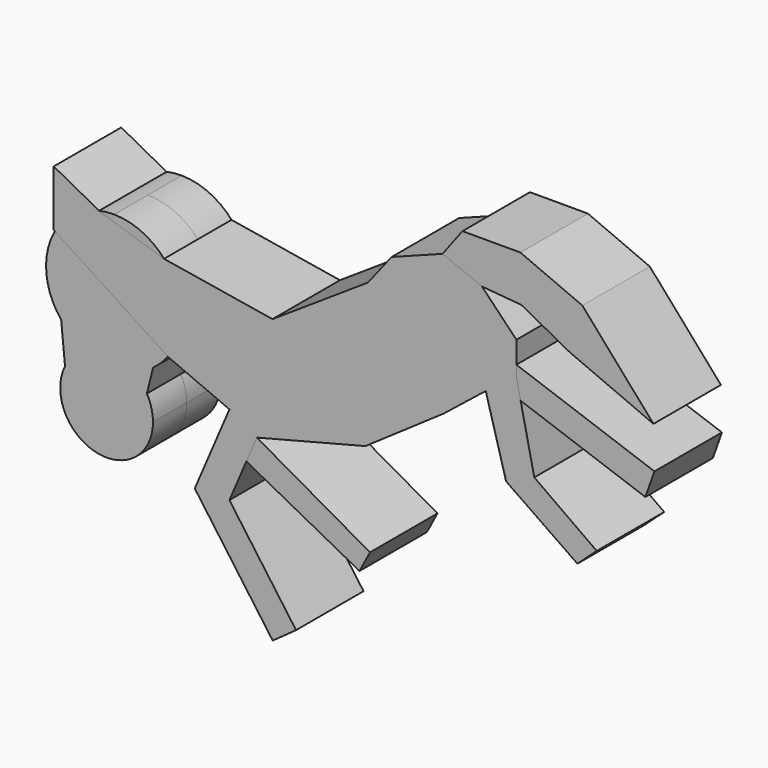
from build123d import *

# Parameters (mm, degrees)
F0_W        = 150.6141573191
F0_H        = 79.405464232
F1_DEPTH    = 63.5
F2_T1_DEPTH = 658.6141573191
F3_T1_DEPTH = 718.5752538832
F7_DEPTH    = 12.7
F9_DEPTH    = 12.7
F10_DEPTH   = 12.7


# Not quite as in the source:
# - a fillet or chamfer that OpenCascade refuses, or shapes differently, is made with other operations: its cross-section is extruded or revolved along the edge and cut away or added


with BuildPart() as f1:
    # F0 (on Front) → F1 (new body, symmetric)
    with BuildSketch(Plane.XZ):
        with Locations((-10.1514682174, 0)):
            Rectangle(F0_W, F0_H)
    extrude(amount=F1_DEPTH, both=True)

    # F2: fillet of radius 101.6 on 2 edges, made by hand

    # F2_s2 → F2_t1 (cut)
    with BuildSketch(Plane.YZ.offset(-339.4585468769)):
        with BuildLine():
            ThreePointArc((-38.1, -39.702732116), (33.7420489686, -9.9447810845), (63.5, 61.897267884))
            Line((63.5, 61.897267884), (63.5, -39.702732116))
            Line((63.5, -39.702732116), (-38.1, -39.702732116))
        make_face()
        with BuildLine():
            ThreePointArc((38.1, -39.702732116), (-33.7420489686, -9.9447810845), (-63.5, 61.897267884))
            Line((-63.5, 61.897267884), (-63.5, -39.702732116))
            Line((-63.5, -39.702732116), (38.1, -39.702732116))
        make_face()
    extrude(amount=F2_T1_DEPTH, mode=Mode.SUBTRACT)

    # F3: fillet of radius 63.5 on 1 edges, made by hand

    # F3_s2 → F3_t1 (cut)
    with BuildSketch(Plane.YZ.offset(-369.439095159)):
        with BuildLine():
            ThreePointArc((-63.5, 61.8972269458), (0, -1.6027474678), (63.5, 61.8972269458))
            ThreePointArc((63.5, 61.8972269458), (46.1422582324, 5.1011242834), (0, -32.2884529021))
            ThreePointArc((0, -32.2884529021), (-46.1422582324, 5.1011242834), (-63.5, 61.8972269458))
        make_face()
    extrude(amount=F3_T1_DEPTH, mode=Mode.SUBTRACT)


with BuildPart() as f1b:
    # F0 (on Front) → F1, piece 2 (new body, symmetric)
    with BuildSketch(Plane.XZ):
        Polygon((31.3350483775, 122.2248598933), (31.3350483775, 93.6296462137), (77.3309990764, 97.4231287837), (73.4557332426, 72.6213976741), (123.3269497752, 72.6213976741), (123.3269497752, 122.2248598933), align=None)
        Polygon((77.3309990764, 97.4231287837), (31.3350483775, 93.6296462137), (31.3350483775, 72.6213976741), (73.4557332426, 72.6213976741), align=None)
    extrude(amount=F1_DEPTH, both=True)


with BuildPart() as f7:
    # F6 (on Front) → F7 (new body, symmetric)
    with BuildSketch(Plane.XZ):
        with BuildLine():
            ThreePointArc((-36.6087691493, 35.5593333212), (-32.619344121, 34.8654693263), (-28.9966608866, 33.0562912025))
            ThreePointArc((-28.9966608866, 33.0562912025), (-25.8689313613, 34.2954979773), (-22.9885519546, 36.0338132212))
            Line((-22.9885519546, 36.0338132212), (-16.6514110853, 61.4541698217))
            ThreePointArc((-16.6514110853, 61.4541698217), (-24.0542736375, 69.6886763572), (-34.6755571583, 72.818821437))
            Line((-34.6755571583, 72.818821437), (-36.6087691493, 35.5593333212))
        make_face()
        with BuildLine():
            ThreePointArc((-43.3512285275, 34.0273458631), (-40.0763049725, 35.2171943654), (-36.6087691493, 35.5593333212))
            Line((-36.6087691493, 35.5593333212), (-34.6755571583, 72.818821437))
            ThreePointArc((-34.6755571583, 72.818821437), (-45.2570577506, 69.977044348), (-52.8245618349, 62.05386735))
            Line((-52.8245618349, 62.05386735), (-50.6579192972, 39.6844671989))
            ThreePointArc((-50.6579192972, 39.6844671989), (-47.3304404617, 36.4350200118), (-43.3512285275, 34.0273458631))
        make_face()
        with BuildLine():
            ThreePointArc((-48.0856804005, 13.1275062956), (-43.6534019652, 9.3288594795), (-38.0556191372, 7.6736745436))
            Line((-38.0556191372, 7.6736745436), (-36.779418711, 32.2703431094))
            ThreePointArc((-36.779418711, 32.2703431094), (-40.1393756094, 32.8718639323), (-43.3512285275, 34.0273458631))
            ThreePointArc((-43.3512285275, 34.0273458631), (-46.9310511113, 31.3995108928), (-49.5049525713, 27.7807158395))
            Line((-49.5049525713, 27.7807158395), (-48.0856804005, 13.1275062956))
        make_face()
        with BuildLine():
            Line((-29.5321783365, 9.785175307), (-24.8586907719, 28.5320712513))
            ThreePointArc((-24.8586907719, 28.5320712513), (-26.6763399678, 31.0240595915), (-28.9966608866, 33.0562912025))
            ThreePointArc((-28.9966608866, 33.0562912025), (-32.8498609048, 32.2852551832), (-36.779418711, 32.2703431094))
            Line((-36.779418711, 32.2703431094), (-38.0556191372, 7.6736745436))
            ThreePointArc((-38.0556191372, 7.6736745436), (-33.6236322142, 8.0421144346), (-29.5321783365, 9.785175307))
        make_face()
        with BuildLine():
            Line((-16.6514110853, 61.4541698217), (-22.9885519546, 36.0338132212))
            ThreePointArc((-22.9885519546, 36.0338132212), (-16.7985245944, 43.2545420146), (-14.5726177745, 52.5012009711))
            ThreePointArc((-14.5726177745, 52.5012009711), (-15.0991379608, 57.0967703828), (-16.6514110853, 61.4541698217))
        make_face()
        with BuildLine():
            ThreePointArc((-36.779418711, 32.2703431094), (-32.8498609048, 32.2852551832), (-28.9966608866, 33.0562912025))
            ThreePointArc((-28.9966608866, 33.0562912025), (-32.619344121, 34.8654693263), (-36.6087691493, 35.5593333212))
            Line((-36.6087691493, 35.5593333212), (-36.779418711, 32.2703431094))
        make_face()
        with BuildLine():
            ThreePointArc((-52.8245618349, 62.05386735), (-55.1155078554, 50.5423444275), (-50.6579192972, 39.6844671989))
            Line((-50.6579192972, 39.6844671989), (-52.8245618349, 62.05386735))
        make_face()
        with BuildLine():
            Line((-36.779418711, 32.2703431094), (-36.6087691493, 35.5593333212))
            ThreePointArc((-36.6087691493, 35.5593333212), (-40.0763049725, 35.2171943654), (-43.3512285275, 34.0273458631))
            ThreePointArc((-43.3512285275, 34.0273458631), (-40.1393756094, 32.8718639323), (-36.779418711, 32.2703431094))
        make_face()
        with BuildLine():
            ThreePointArc((-49.5049525713, 27.7807158395), (-46.9310511113, 31.3995108928), (-43.3512285275, 34.0273458631))
            ThreePointArc((-43.3512285275, 34.0273458631), (-47.3304404617, 36.4350200118), (-50.6579192972, 39.6844671989))
            Line((-50.6579192972, 39.6844671989), (-49.5049525713, 27.7807158395))
        make_face()
        with BuildLine():
            ThreePointArc((-28.9966608866, 33.0562912025), (-26.6763399678, 31.0240595915), (-24.8586907719, 28.5320712513))
            Line((-24.8586907719, 28.5320712513), (-22.9885519546, 36.0338132212))
            ThreePointArc((-22.9885519546, 36.0338132212), (-25.8689313613, 34.2954979773), (-28.9966608866, 33.0562912025))
        make_face()
        with BuildLine():
            ThreePointArc((-29.5321783365, 9.785175307), (-24.7530043734, 14.8527299858), (-23.0159053765, 21.5983286448))
            ThreePointArc((-23.0159053765, 21.5983286448), (-23.4844617139, 25.1855505694), (-24.8586907719, 28.5320712513))
            Line((-24.8586907719, 28.5320712513), (-29.5321783365, 9.785175307))
        make_face()
        with BuildLine():
            ThreePointArc((-49.5049525713, 27.7807158395), (-50.882832593, 20.251919629), (-48.0856804005, 13.1275062956))
            Line((-48.0856804005, 13.1275062956), (-49.5049525713, 27.7807158395))
        make_face()
    extrude(amount=F7_DEPTH, both=True)


with BuildPart() as f9:
    # F8 (on Front) → F9 (new body, symmetric)
    with BuildSketch(Plane.XZ):
        Polygon((70.1734498143, 102.5099307299), (64.1641393304, 94.530403614), (76.0201886296, 89.753575623), (87.9124104977, 88.7197852135), (102.4909329914, 80.9034005742), (127.6726275682, 70.1168328524), (106.2612786499, 94.530403614), (87.6327380538, 102.5099307299), align=None)
    extrude(amount=F9_DEPTH, both=True)


with BuildPart() as f9b:
    # F8 (on Front) → F9, piece 2 (new body, symmetric)
    with BuildSketch(Plane.XZ):
        Polygon((127.969712019, 57.6258897781), (86.4127874374, 72.3803937435), (86.4127874374, 69.103308022), (87.6771708107, 63.2699279244), (125.2387401997, 49.9339476978), align=None)
    extrude(amount=F9_DEPTH, both=True)


with BuildPart() as f9c:
    # F8 (on Front) → F9, piece 3 (new body, symmetric)
    with BuildSketch(Plane.XZ):
        Polygon((8.2513917411, 27.6518290569), (5.10901674, 20.3158228717), (39.1638986766, 2.32507498), (42.3252065188, 8.309148904), align=None)
    extrude(amount=F9_DEPTH, both=True)


with BuildPart() as f10:
    # F8 (on Front) → F10 (new body, symmetric)
    with BuildSketch(Plane.XZ):
        Polygon((-52.8965368867, 79.6501561999), (-52.8965368867, 62.8078132868), (-18.3518156409, 40.3029546142), (0, 32.4419625103), (-10.4339636263, 8.0834369776), (13.0310822278, -24.6068127453), (20.0616800202, -19.5602529613), (0, 8.388609095), (5.10901674, 20.3158228717), (8.2513917411, 27.6518290569), (40.949832648, 36.0271781683), (64.455486834, 52.2657185793), (77.1777108312, 62.4108165503), (83.3045616746, 40.4580123723), (104.7781407833, 25.6019085646), (110.5931252241, 30.8859813958), (91.7972102761, 44.2616455257), (87.6771708107, 63.2699279244), (86.4127874374, 69.103308022), (86.4127874374, 72.3803937435), (86.4127874374, 79.0046826005), (76.0201886296, 89.753575623), (64.1641393304, 94.530403614), (48.835285008, 88.7197852135), (41.6805818677, 79.5953571796), (12.9594327882, 60.5743080378), (-19.7210758924, 65.9544691443), (-38.7121960521, 72.0541030169), align=None)
    extrude(amount=F10_DEPTH, both=True)


solid = Compound([f7.part, f9.part, f9b.part, f9c.part, f10.part])
